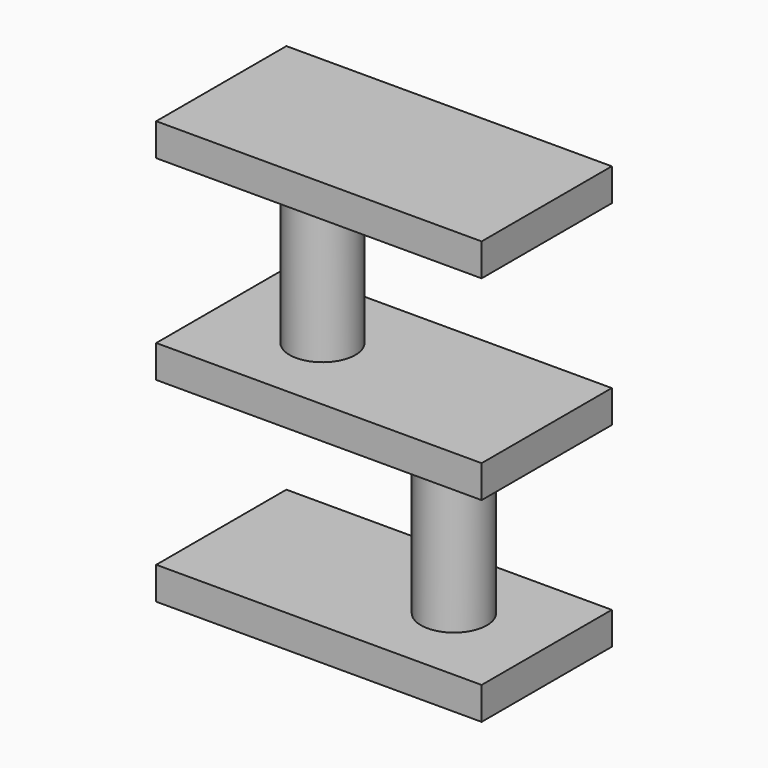
from build123d import *

# Parameters (mm, degrees)
F1_DEPTH = 25
F2_DEPTH = 25
F3_DEPTH = 25
F4_R     = 5.0692688019
F5_DEPTH = 27.5
F4_R_2   = 5.0566520552
F6_DEPTH = 27.5


with BuildPart() as f1:
    # F0 (on Front) → F1 (new body)
    with BuildSketch(Plane.XZ):
        Polygon((0, -27.5), (0, -32.5), (50, -32.5), (50, -27.5), (5, -27.5), align=None)
    extrude(amount=F1_DEPTH)

    # F4 (on Top) → F5 (join, through all)
    with BuildSketch(Plane.XY):
        with Locations((35.7477681773, -12.5000000002)):
            Circle(F4_R)
    extrude(amount=-F5_DEPTH)


with BuildPart() as f2:
    # F0 (on Front) → F2 (new body, through all)
    with BuildSketch(Plane.XZ):
        Polygon((0, 2.5), (0, -2.5), (5, -2.5), (50, -2.5), (50, 2.5), (5, 2.5), align=None)
    extrude(amount=F2_DEPTH)


with BuildPart() as f3:
    # F0 (on Front) → F3 (new body, through all)
    with BuildSketch(Plane.XZ):
        Polygon((0, 32.5), (0, 27.5), (5, 27.5), (50, 27.5), (50, 32.5), align=None)
    extrude(amount=F3_DEPTH)

    # F4 (on Top) → F6 (join, through all)
    with BuildSketch(Plane.XY):
        with Locations((15.5519776108, -12.5000000002)):
            Circle(F4_R_2)
    extrude(amount=F6_DEPTH)


solid = Compound([f1.part, f2.part, f3.part])
